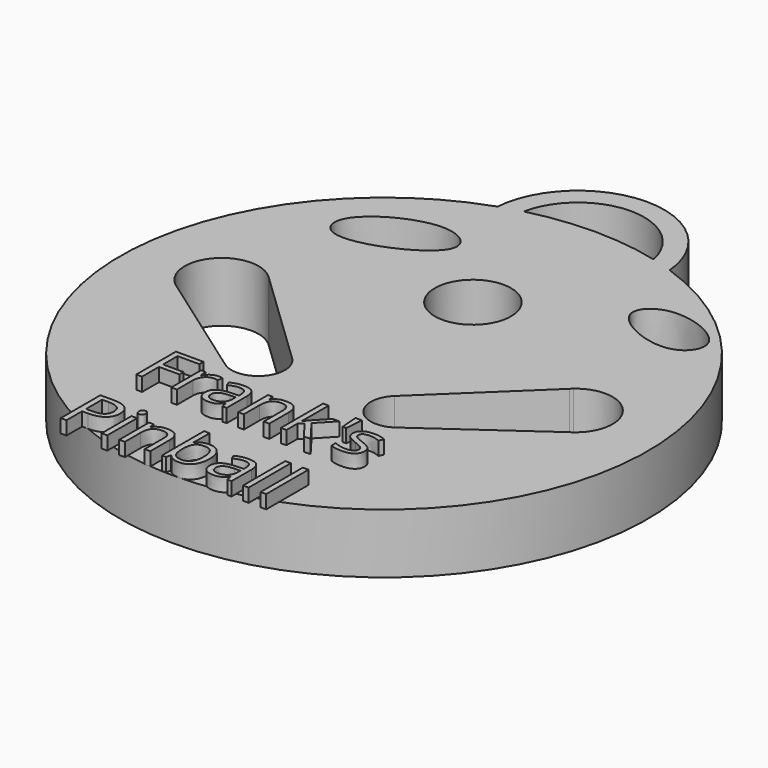
from build123d import *

# Parameters (mm, degrees)
F0_R         = 10.0506199241
F1_DEPTH     = 15.748
F2_TEXT_SIZE = 18.305124508
F3_DEPTH     = 3.556


# Not quite as in the source:
# - Text() gives the source's letters only with a copy of the font that has no kerning and outlines rounded to 1/6400 em; it was checked with that copy


with BuildPart() as f1:
    # F0 (on Top) → F1 (new body)
    with BuildSketch(Plane.XY):
        with BuildLine():
            ThreePointArc((-22.6848959163, 65.7553812639), (0, -69.5584262897), (22.6848959163, 65.7553812639))
            ThreePointArc((22.6848959163, 65.7553812639), (0, 86.6445640898), (-22.6848959163, 65.7553812639))
        make_face()
        with BuildLine():
            ThreePointArc((-52.6735718937, -2.8356859106), (-54.126387688, 11.0377459491), (-40.2207272532, 12.1401946653))
            ThreePointArc((-40.2207272532, 12.1401946653), (-39.903285642, 11.8497710582), (-39.5989774937, 11.5456138637))
            Line((-39.5989774937, 11.5456138637), (-13.4946921554, -13.4179774567))
            ThreePointArc((-13.4946921554, -13.4179774567), (-12.9290843268, -22.9907056018), (-22.4346003688, -24.2564864401))
            Line((-22.4346003688, -24.2564864401), (-51.8453802756, -3.4223635176))
            ThreePointArc((-51.8453802756, -3.4223635176), (-52.2671217282, -3.1398177933), (-52.6735718937, -2.8356859106))
        make_face(mode=Mode.SUBTRACT)
        with BuildLine():
            ThreePointArc((22.4346003688, -24.2564864401), (12.9290843268, -22.9907056018), (13.4946921554, -13.4179774567))
            Line((13.4946921554, -13.4179774567), (39.5989774937, 11.5456138637))
            ThreePointArc((39.5989774937, 11.5456138637), (39.903285642, 11.8497710582), (40.2207272532, 12.1401946653))
            ThreePointArc((40.2207272532, 12.1401946653), (54.126387688, 11.0377459491), (52.6735718937, -2.8356859106))
            ThreePointArc((52.6735718937, -2.8356859106), (52.2671217282, -3.1398177933), (51.8453802756, -3.4223635176))
            Line((51.8453802756, -3.4223635176), (22.4346003688, -24.2564864401))
        make_face(mode=Mode.SUBTRACT)
        with BuildLine():
            add(Edge.make_bspline(
                [(-24.6028024703, 51.4707304537), (-31.4524390225, 52.0764449834), (-47.2626468135, 43.8814068488), (-42.1610783573, 30.6543984207), (-11.9918427181, 43.739577277), (-20.2270904618, 51.0837854938), (-24.6028024703, 51.4707304537)],
                knots=[0, 0, 0, 0, 0.3044818826, 0.480868386, 0.8054896753, 1, 1, 1, 1], degree=3))
        make_face(mode=Mode.SUBTRACT)
        with Locations((0, 29.2932782322)):
            Circle(F0_R, mode=Mode.SUBTRACT)
        with BuildLine():
            add(Edge.make_bspline(
                [(34.2662259936, 51.4707304537), (39.7329606939, 52.3857372806), (53.4329080582, 46.8778835572), (44.9063310165, 34.5078071648), (23.906545079, 44.0562904681), (30.3320462202, 50.8122384017), (34.2662259936, 51.4707304537)],
                knots=[0, 0, 0, 0, 0.2882733869, 0.4970571581, 0.7925417292, 1, 1, 1, 1], degree=3))
        make_face(mode=Mode.SUBTRACT)
        with BuildLine():
            ThreePointArc((-17.1014588037, 67.4233993112), (0, 81.3466760282), (17.1014588037, 67.4233993112))
            ThreePointArc((17.1014588037, 67.4233993112), (0, 69.5584262897), (-17.1014588037, 67.4233993112))
        make_face(mode=Mode.SUBTRACT)
    extrude(amount=F1_DEPTH)

    # F2 (on face) → F3 (join)
    with BuildSketch(Plane.XY.offset(15.748)):
        with Locations((-31.5164001659, -44.4823075086)):
            Text("Frank's", F2_TEXT_SIZE, font='Open Sans', text_align=(TextAlign.LEFT, TextAlign.BOTTOM))
        with Locations((-31.5164001659, -69.3772768395)):
            Text('Pinball', F2_TEXT_SIZE, font='Open Sans', text_align=(TextAlign.LEFT, TextAlign.BOTTOM))
    extrude(amount=F3_DEPTH)


solid = f1.part
